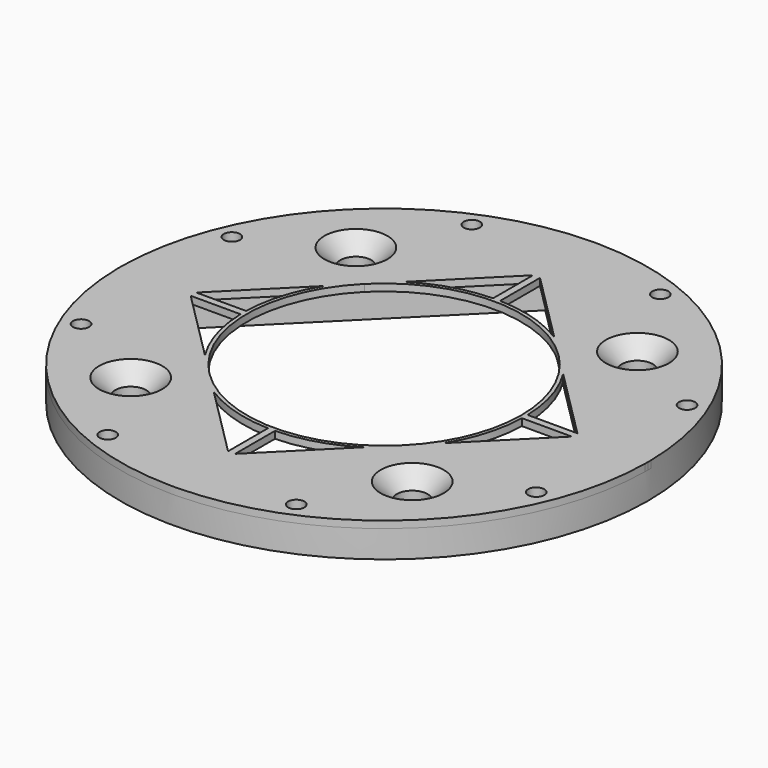
from build123d import *

# Parameters (mm, degrees)
F0_R           = 37.5
F1_DEPTH       = 3.86
F3_DEPTH       = 1
F5_D           = 4.4
F5_DEPTH       = 50
F5_CSINK_D     = 8.96
F5_CSINK_ANGLE = 90
F5_TIP         = 1.3218933619
F6_D           = 2.3
F6_DEPTH       = 50
F6_TIP         = 0.6909897119


# Not quite as in the source:
# - a feature names something its author has since deleted; it is built from what else it names


with BuildPart() as f1:
    # F0 (on Top) → F1 (new body)
    with BuildSketch(Plane.XY):
        Circle(F0_R)
        with BuildLine():
            Line((35.5279936079, -6.7726684482), (33.9669435175, -8.4407788788))
            ThreePointArc((33.9669435175, -8.4407788788), (24.9465264027, -24.5493547866), (8.9847812304, -33.8271149559))
            Line((8.9847812304, -33.8271149559), (7.0870357741, -35.7248604122))
            Line((7.0870357741, -35.7248604122), (5.8669428771, -34.5047675152))
            Line((5.8669428771, -34.5047675152), (2.7425574301, -31.3803820681))
            ThreePointArc((2.7425574301, -31.3803820681), (-22.2891525488, 22.2585641643), (31.3841187925, -2.6994606157))
            Line((31.3841187925, -2.6994606157), (34.5192493346, -5.7811266526))
            Line((34.5192493346, -5.7811266526), (35.5279936079, -6.7726684482))
        make_face(mode=Mode.SUBTRACT)
        with BuildLine():
            Line((28.6378246381, 0), (31.3841187925, -2.6994606157))
            ThreePointArc((31.3841187925, -2.6994606157), (-22.2891525488, 22.2585641643), (2.7425574301, -31.3803820681))
            Line((2.7425574301, -31.3803820681), (0, -28.6378246381))
            Line((0, -28.6378246381), (-28.6378246381, 0))
            Line((-28.6378246381, 0), (0, 28.6378246381))
            Line((0, 28.6378246381), (28.6378246381, 0))
        make_face()
        with BuildLine():
            Line((30.967620581, -5.7668427717), (26.7850823006, -1.8527423374))
            Line((26.7850823006, -1.8527423374), (1.8586698278, -26.7791548102))
            Line((1.8586698278, -26.7791548102), (6.2368967636, -30.8763844833))
            ThreePointArc((6.2368967636, -30.8763844833), (22.442510977, -22.1039295386), (30.967620581, -5.7668427717))
        make_face()
        with BuildLine():
            Line((33.9006451973, -8.5116240875), (30.967620581, -5.7668427717))
            ThreePointArc((30.967620581, -5.7668427717), (22.442510977, -22.1039295386), (6.2368967636, -30.8763844833))
            Line((6.2368967636, -30.8763844833), (9.1806708369, -33.6312253494))
            Line((9.1806708369, -33.6312253494), (8.9847812304, -33.8271149559))
            ThreePointArc((8.9847812304, -33.8271149559), (24.9465264027, -24.5493547866), (33.9669435175, -8.4407788788))
            Line((33.9669435175, -8.4407788788), (33.9006451973, -8.5116240875))
        make_face()
    extrude(amount=F1_DEPTH)

    # F2 (on face) → F3 (join)
    with BuildSketch(Plane.XY.offset(3.86)):
        with BuildLine():
            ThreePointArc((37.4966665185, -0.5), (37.4991666204, -0.250005556), (37.5, 0))
            ThreePointArc((37.5, 0), (37.4991666204, 0.250005556), (37.4966665185, 0.5))
            Line((37.4966665185, 0.5), (37.4966665185, -0.5))
        make_face()
        with BuildLine():
            Line((37.4966665185, -0.5), (37.4966665185, 0.5))
            ThreePointArc((37.4966665185, 0.5), (26.5165042945, 26.5165042945), (0.5, 37.4966665185))
            Line((0.5, 37.4966665185), (-0.5, 37.4966665185))
            ThreePointArc((-0.5, 37.4966665185), (-26.5165042945, 26.5165042945), (-37.4966665185, 0.5))
            Line((-37.4966665185, 0.5), (-37.4966665185, -0.5))
            ThreePointArc((-37.4966665185, -0.5), (-26.5165042945, -26.5165042945), (-0.5, -37.4966665185))
            Line((-0.5, -37.4966665185), (0.5, -37.4966665185))
            ThreePointArc((0.5, -37.4966665185), (26.5165042945, -26.5165042945), (37.4966665185, -0.5))
        make_face()
        with BuildLine():
            Line((-0.5, -27.0771644663), (-10.6461309606, -16.9310335056))
            ThreePointArc((-10.6461309606, -16.9310335056), (-5.7796293509, -19.1466938286), (-0.5, -19.9937490231))
            Line((-0.5, -19.9937490231), (-0.5, -27.0771644663))
        make_face(mode=Mode.SUBTRACT)
        with BuildLine():
            ThreePointArc((-19.9937490231, -0.5), (-19.1466938286, -5.7796293509), (-16.9310335056, -10.6461309606))
            Line((-16.9310335056, -10.6461309606), (-27.0771644663, -0.5))
            Line((-27.0771644663, -0.5), (-19.9937490231, -0.5))
        make_face(mode=Mode.SUBTRACT)
        with BuildLine():
            ThreePointArc((0.5, -19.9937490231), (5.7796293509, -19.1466938286), (10.6461309606, -16.9310335056))
            Line((10.6461309606, -16.9310335056), (0.5, -27.0771644663))
            Line((0.5, -27.0771644663), (0.5, -19.9937490231))
        make_face(mode=Mode.SUBTRACT)
        with BuildLine():
            Line((27.0771644663, -0.5), (16.9310335056, -10.6461309606))
            ThreePointArc((16.9310335056, -10.6461309606), (19.1466938286, -5.7796293509), (19.9937490231, -0.5))
            Line((19.9937490231, -0.5), (27.0771644663, -0.5))
        make_face(mode=Mode.SUBTRACT)
        with BuildLine():
            Line((-27.0771644663, 0.5), (-16.9310335056, 10.6461309606))
            ThreePointArc((-16.9310335056, 10.6461309606), (-19.1466938286, 5.7796293509), (-19.9937490231, 0.5))
            Line((-19.9937490231, 0.5), (-27.0771644663, 0.5))
        make_face(mode=Mode.SUBTRACT)
        with BuildLine():
            ThreePointArc((-0.5, 19.9937490231), (-5.7796293509, 19.1466938286), (-10.6461309606, 16.9310335056))
            Line((-10.6461309606, 16.9310335056), (-0.5, 27.0771644663))
            Line((-0.5, 27.0771644663), (-0.5, 19.9937490231))
        make_face(mode=Mode.SUBTRACT)
        with BuildLine():
            ThreePointArc((13.7885822494, 13.7885822168), (18.0156508884, 7.4623269205), (19.5, 0))
            ThreePointArc((19.5, 0), (18.015650884, -7.4623269311), (13.7885822331, -13.7885822331))
            ThreePointArc((13.7885822331, -13.7885822331), (4.88e-08, -19.5), (-13.7885821641, -13.7885823022))
            ThreePointArc((-13.7885821641, -13.7885823022), (-19.5, -3.62e-08), (-13.7885822154, 13.7885822509))
            ThreePointArc((-13.7885822154, 13.7885822509), (2.41e-08, 19.5), (13.7885822494, 13.7885822168))
        make_face(mode=Mode.SUBTRACT)
        with BuildLine():
            ThreePointArc((19.9937490231, 0.5), (19.1466938286, 5.7796293509), (16.9310335056, 10.6461309606))
            Line((16.9310335056, 10.6461309606), (27.0771644663, 0.5))
            Line((27.0771644663, 0.5), (19.9937490231, 0.5))
        make_face(mode=Mode.SUBTRACT)
        with BuildLine():
            Line((0.5, 27.0771644663), (10.6461309606, 16.9310335056))
            ThreePointArc((10.6461309606, 16.9310335056), (5.7796293509, 19.1466938286), (0.5, 19.9937490231))
            Line((0.5, 19.9937490231), (0.5, 27.0771644663))
        make_face(mode=Mode.SUBTRACT)
        with BuildLine():
            Line((-0.5, 37.4966665185), (0.5, 37.4966665185))
            ThreePointArc((0.5, 37.4966665185), (0, 37.5), (-0.5, 37.4966665185))
        make_face()
        with BuildLine():
            ThreePointArc((-0.5, -37.4966665185), (0, -37.5), (0.5, -37.4966665185))
            Line((0.5, -37.4966665185), (-0.5, -37.4966665185))
        make_face()
        with BuildLine():
            Line((-37.4966665185, -0.5), (-37.4966665185, 0.5))
            ThreePointArc((-37.4966665185, 0.5), (-37.5, 0), (-37.4966665185, -0.5))
        make_face()
    extrude(amount=F3_DEPTH)

    # F5
    with Locations(Plane.XY.offset(4.86)):
        with Locations((-20, -20), (20, -20), (20, 20), (-20, 20)):
            CounterSinkHole(F5_D / 2, F5_CSINK_D / 2, depth=F5_DEPTH, counter_sink_angle=F5_CSINK_ANGLE)
            with Locations((0, 0, -(F5_DEPTH + F5_TIP / 2))):  # 118° drill point
                Cone(0, F5_D / 2, F5_TIP, mode=Mode.SUBTRACT)

    # F6
    with Locations(Plane(origin=(0, 0, 0), x_dir=(1, 0, 0), z_dir=(0, 0, -1))):
        with Locations((-32.3357836379, -13.3939201328), (-13.3939201328, -32.3357836379), (13.3939201328, -32.3357836379), (32.3357836379, -13.3939201328), (32.3357836379, 13.3939201328), (13.3939201328, 32.3357836379), (-13.3939201328, 32.3357836379), (-32.3357836379, 13.3939201328)):
            Hole(F6_D / 2, depth=F6_DEPTH)
            with Locations((0, 0, -(F6_DEPTH + F6_TIP / 2))):  # 118° drill point
                Cone(0, F6_D / 2, F6_TIP, mode=Mode.SUBTRACT)


solid = f1.part
